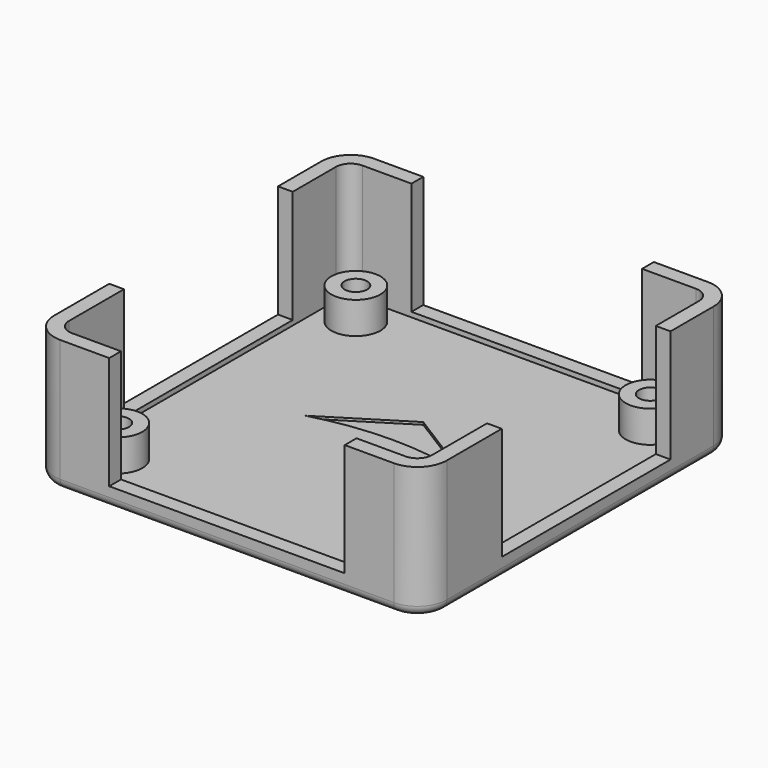
from build123d import *

# Parameters (mm, degrees)
F0_W          = 40
F0_H          = 40
F1_DEPTH      = 1.5
F2_W          = 40
F2_H          = 40
F2_W_2        = 37
F2_H_2        = 37
F3_DEPTH      = 12
F4_R          = 2.5
F5_DEPTH      = 3.25
F6_R          = 1.15
F7_DEPTH      = 4.751
F9_DEPTH      = 11.5
F11_DEPTH     = 0.25
F12_R         = 1
F13_T1_DEPTH  = 21
F13_T4_ANGLE  = 90
F13_T6_ANGLE  = 90
F13_T8_ANGLE  = 90
F13_T10_ANGLE = 90
F14_R         = 1.5


# Not quite as in the source:
# - a fillet or chamfer that OpenCascade refuses, or shapes differently, is made with other operations: its cross-section is extruded or revolved along the edge and cut away or added


with BuildPart() as f1:
    # F0 (on Top) → F1 (new body)
    with BuildSketch(Plane.XY):
        Rectangle(F0_W, F0_H)
    extrude(amount=F1_DEPTH)

    # F2 (on face) → F3 (join)
    with BuildSketch(Plane.XY.offset(1.5)):
        Rectangle(F2_W, F2_H)
        Rectangle(F2_W_2, F2_H_2, mode=Mode.SUBTRACT)
    extrude(amount=F3_DEPTH)

    # F4 (on face) → F5 (join)
    with BuildSketch(Plane.XY.offset(1.5)):
        with Locations((-15, 15.1671093126)):
            Circle(F4_R)
        with Locations((15, 15.1671093126)):
            Circle(F4_R)
        with Locations((15, -15.1671093126)):
            Circle(F4_R)
        with Locations((-15, -15.1671093126)):
            Circle(F4_R)
    extrude(amount=F5_DEPTH)

    # F6 (on face) → F7 (cut, through all)
    with BuildSketch(Plane.XY.offset(4.75)):
        with Locations((-15, 15.1671093126)):
            Circle(F6_R)
        with Locations((15, 15.1671093126)):
            Circle(F6_R)
        with Locations((-15, -15.1671093126)):
            Circle(F6_R)
        with Locations((15, -15.1671093126)):
            Circle(F6_R)
    extrude(amount=-F7_DEPTH, mode=Mode.SUBTRACT)

    # F8 (on face) → F9 (cut)
    with BuildSketch(Plane.XY.offset(13.5)):
        Polygon((11.5, 25.4), (-12, 25.4), (-12, 11.5), (-27.1345967194, 11.5), (-27.1345967194, -10), (-12, -10), (-12, -25.4), (12, -25.4), (12, -10), (25.4, -10), (25.4, 11.5), (11.5, 11.5), align=None)
    extrude(amount=-F9_DEPTH, mode=Mode.SUBTRACT)

    # F10 (on face) → F11 (cut)
    with BuildSketch(Plane.XY.offset(1.5)):
        with BuildLine():
            Line((8, 0), (0, 5))
            Line((0, 5), (-8, 0))
            ThreePointArc((-8, 0), (0, 1.0863354104), (8, 0))
        make_face()
    extrude(amount=-F11_DEPTH, mode=Mode.SUBTRACT)

    # F12
    f12_edges = [f1.edges().sort_by_distance(p)[0] for p in [
        (20, 0, 0),
        (0, -20, 0),
        (0, 20, 0),
        (-20, 0, 0),
        (-16.15, -15.167109, 0),
        (13.85, -15.167109, 0),
        (-16.15, 15.167109, 0),
        (13.85, 15.167109, 0),
    ]]
    fillet(f12_edges, radius=F12_R)

    # F13: fillet of radius 3 on 4 edges, made by hand

    # F13_s2 → F13_t1 (cut)
    with BuildSketch(Plane.XY):
        with BuildLine():
            ThreePointArc((20, -17), (19.1213203436, -19.1213203436), (17, -20))
            Line((17, -20), (20, -20))
            Line((20, -20), (20, -17))
        make_face()
        with BuildLine():
            ThreePointArc((20, 17), (19.1213203436, 19.1213203436), (17, 20))
            Line((17, 20), (20, 20))
            Line((20, 20), (20, 17))
        make_face()
        with BuildLine():
            ThreePointArc((-17, 20), (-19.1213203436, 19.1213203436), (-20, 17))
            Line((-20, 17), (-20, 20))
            Line((-20, 20), (-17, 20))
        make_face()
        with BuildLine():
            ThreePointArc((-17, -20), (-19.1213203436, -19.1213203436), (-20, -17))
            Line((-20, -17), (-20, -20))
            Line((-20, -20), (-17, -20))
        make_face()
    extrude(amount=F13_T1_DEPTH, mode=Mode.SUBTRACT)

    # F13_s3 → F13_t4 (revolve, cut)
    with BuildSketch(Plane.YZ.offset(-17)):
        with BuildLine():
            ThreePointArc((-19, 0), (-19.7071067812, 0.2928932188), (-20, 1))
            Line((-20, 1), (-20, 0))
            Line((-20, 0), (-19, 0))
        make_face()
    revolve(axis=Axis((-17, -17, 0), (0, 0, -1)), revolution_arc=F13_T4_ANGLE, mode=Mode.SUBTRACT)

    # F13_s5 → F13_t6 (revolve, cut)
    with BuildSketch(Plane.XZ.offset(-17)):
        with BuildLine():
            ThreePointArc((-19, 0), (-19.7071067812, 0.2928932188), (-20, 1))
            Line((-20, 1), (-20, 0))
            Line((-20, 0), (-19, 0))
        make_face()
    revolve(axis=Axis((-17, 17, 0), (0, 0, -1)), revolution_arc=F13_T6_ANGLE, mode=Mode.SUBTRACT)

    # F13_s7 → F13_t8 (revolve, cut)
    with BuildSketch(Plane.YZ.offset(17)):
        with BuildLine():
            ThreePointArc((19, 0), (19.7071067812, 0.2928932188), (20, 1))
            Line((20, 1), (20, 0))
            Line((20, 0), (19, 0))
        make_face()
    revolve(axis=Axis((17, 17, 0), (0, 0, -1)), revolution_arc=F13_T8_ANGLE, mode=Mode.SUBTRACT)

    # F13_s9 → F13_t10 (revolve, cut)
    with BuildSketch(Plane.XZ.offset(17)):
        with BuildLine():
            ThreePointArc((19, 0), (19.7071067812, 0.2928932188), (20, 1))
            Line((20, 1), (20, 0))
            Line((20, 0), (19, 0))
        make_face()
    revolve(axis=Axis((17, -17, 0), (0, 0, -1)), revolution_arc=F13_T10_ANGLE, mode=Mode.SUBTRACT)

    # F14
    f14_edges = [f1.edges().sort_by_distance(p)[0] for p in [
        (-18.5, 18.5, 7.5),
        (18.5, 18.5, 7.5),
        (-18.5, -18.5, 7.5),
        (18.5, -18.5, 7.5),
    ]]
    fillet(f14_edges, radius=F14_R)


solid = f1.part
